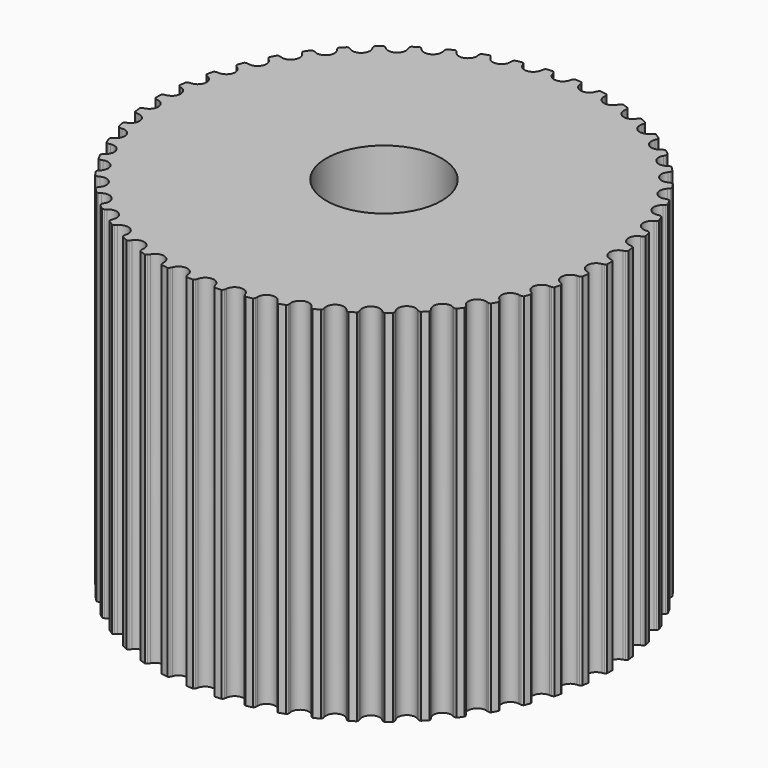
from build123d import *

# Parameters (mm, degrees)
F0_R     = 4
F1_DEPTH = 25


# Not quite as in the source:
# - ends of sketch curves that miss each other by under 0.0002 mm in the source are joined


with BuildPart() as f1:
    # F0 (on Top) → F1 (new body)
    with BuildSketch(Plane.XY):
        with BuildLine():
            ThreePointArc((5.0538548701, 14.8313976165), (4.8338819161, 14.9042559245), (4.6129350386, 14.9741051251))
            ThreePointArc((4.6129350386, 14.9741051251), (4.5441993324, 14.946267968), (4.4878171315, 14.8980958886))
            ThreePointArc((4.4878171315, 14.8980958886), (4.4420209944, 14.8370934455), (4.4036843047, 14.7711473513))
            ThreePointArc((4.4036843047, 14.7711473513), (3.7022053294, 14.453002295), (3.2407613785, 15.0697349868))
            ThreePointArc((3.2407613785, 15.0697349868), (3.2389362265, 15.1459926578), (3.2281934751, 15.2215118936))
            ThreePointArc((3.2281934751, 15.2215118936), (3.201998612, 15.2906625624), (3.1551368112, 15.3478637858))
            ThreePointArc((3.1551368112, 15.3478637858), (2.9277664974, 15.3925774546), (2.699806991, 15.4341839489))
            ThreePointArc((2.699806991, 15.4341839489), (2.6351025722, 15.3979510096), (2.5852026476, 15.3430922294))
            ThreePointArc((2.5852026476, 15.3430922294), (2.5474139332, 15.2768308289), (2.5176449061, 15.2066000335))
            ThreePointArc((2.5176449061, 15.2066000335), (1.8615708966, 14.8030459697), (1.3264687832, 15.3570810714))
            ThreePointArc((1.3264687832, 15.3570810714), (1.315100082, 15.432508655), (1.2949769217, 15.5060859735))
            ThreePointArc((1.2949769217, 15.5060859735), (1.2603213274, 15.5714077424), (1.2066603566, 15.622284525))
            ThreePointArc((1.2066603566, 15.622284525), (0.9754784824, 15.6381481518), (0.7441019834, 15.6508556551))
            ThreePointArc((0.7441019834, 15.6508556551), (0.684448921, 15.6067992893), (0.6418182175, 15.5461188946))
            ThreePointArc((0.6418182175, 15.5461188946), (0.6126318129, 15.4756440547), (0.5918997543, 15.4022360541))
            ThreePointArc((0.5918997543, 15.4022360541), (-0.008422, 14.919636), (-0.6087438986, 15.4022360223))
            ThreePointArc((-0.6087438986, 15.4022360223), (-0.6294758129, 15.4756440547), (-0.6586618609, 15.5461190674))
            ThreePointArc((-0.6586618609, 15.5461190674), (-0.7012312489, 15.6065826918), (-0.7608459985, 15.6503330029))
            ThreePointArc((-0.7608459985, 15.6503330029), (-0.9921926068, 15.6370972346), (-1.2233370313, 15.6207054025))
            ThreePointArc((-1.2233370313, 15.6207054025), (-1.2769989996, 15.569519629), (-1.3116886862, 15.5039742317))
            ThreePointArc((-1.3116886862, 15.5039742317), (-1.33181118, 15.4303971915), (-1.3431793008, 15.3549700274))
            ThreePointArc((-1.3431793008, 15.3549700274), (-1.8782818966, 14.8009349697), (-2.5343560792, 15.2044889718))
            ThreePointArc((-2.5343560792, 15.2044889718), (-2.5641249332, 15.2747198289), (-2.6019136975, 15.3409811969))
            ThreePointArc((-2.6019136975, 15.3409811969), (-2.6517255298, 15.3956328998), (-2.7163538339, 15.4315664618))
            ThreePointArc((-2.7163538339, 15.4315664618), (-2.9442174772, 15.3894389341), (-3.1714848475, 15.3442062603))
            ThreePointArc((-3.1714848475, 15.3442062603), (-3.2183068506, 15.2866986193), (-3.2445078833, 15.2173229763))
            ThreePointArc((-3.2445078833, 15.2173229763), (-3.2552512183, 15.1418037568), (-3.2570761686, 15.0655459941))
            ThreePointArc((-3.2570761686, 15.0655459941), (-3.7185201109, 14.4488133511), (-4.4199997516, 14.7669576202))
            ThreePointArc((-4.4199997516, 14.7669576202), (-4.4583356914, 14.8329039882), (-4.504131298, 14.8939067477))
            ThreePointArc((-4.504131298, 14.8939067477), (-4.5603999736, 14.9418840659), (-4.6290219304, 14.9694343117))
            ThreePointArc((-4.6290219304, 14.9694343117), (-4.8498095032, 14.8990807668), (-5.0696161514, 14.8257204436))
            ThreePointArc((-5.0696161514, 14.8257204436), (-5.1088617324, 14.7627975058), (-5.1261608376, 14.6906849879))
            ThreePointArc((-5.1261608376, 14.6906849879), (-5.1273535974, 14.6144149758), (-5.1196065751, 14.5385300687))
            ThreePointArc((-5.1196065751, 14.5385300687), (-5.5001148623, 13.8688261233), (-6.2359372486, 14.0965428322))
            ThreePointArc((-6.2359372486, 14.0965428322), (-6.2822362135, 14.1571640234), (-6.3353161345, 14.2119458535))
            ThreePointArc((-6.3353161345, 14.2119458535), (-6.3971546722, 14.2524927401), (-6.4686889983, 14.2712250176))
            ThreePointArc((-6.4686889983, 14.2712250176), (-6.6789174057, 14.1737545132), (-6.8877958964, 14.0734237881))
            ThreePointArc((-6.8877958964, 14.0734237881), (-6.918845823, 14.0060783452), (-6.9269704732, 13.9323659757))
            ThreePointArc((-6.9269704732, 13.9323659757), (-6.9185946899, 13.856547756), (-6.9013977373, 13.7822320773))
            ThreePointArc((-6.9013977373, 13.7822320773), (-7.1949697757, 13.0701187417), (-7.9535304625, 13.203817595))
            ThreePointArc((-7.9535304625, 13.203817595), (-8.00706254, 13.2581577974), (-8.0665899904, 13.3058550135))
            ThreePointArc((-8.0665899904, 13.3058550135), (-8.1330222057, 13.3383321973), (-8.2063400351, 13.3479511062))
            ThreePointArc((-8.2063400351, 13.3479511062), (-8.402694302, 13.2248996356), (-8.5973508141, 13.0991807164))
            ThreePointArc((-8.5973508141, 13.0991807164), (-8.6197156177, 13.0284751976), (-8.6185378436, 12.954326028))
            ThreePointArc((-8.6185378436, 12.954326028), (-8.6007257896, 12.8801553087), (-8.5743502072, 12.8085809095))
            ThreePointArc((-8.5743502072, 12.8085809095), (-8.7763549932, 12.0652885559), (-9.5456911317, 12.1028598516))
            ThreePointArc((-9.5456911317, 12.1028598516), (-9.6056123132, 12.1500616883), (-9.6706484989, 12.1899220673))
            ThreePointArc((-9.6706484989, 12.1899220673), (-9.740627088, 12.213816696), (-9.814571967, 12.214170792))
            ThreePointArc((-9.814571967, 12.214170792), (-9.9939559602, 12.0674808947), (-10.171321105, 11.9183561232))
            ThreePointArc((-10.171321105, 11.9183561232), (-10.1846477481, 11.8454047013), (-10.174185817, 11.7719877449))
            ThreePointArc((-10.174185817, 11.7719877449), (-10.1472175675, 11.7006345891), (-10.1120794197, 11.6329303458))
            ThreePointArc((-10.1120794197, 11.6329303458), (-10.219332575, 10.8701815734), (-10.9873108533, 10.8110332144))
            ThreePointArc((-10.9873108533, 10.8110332144), (-11.0526756486, 10.8503529134), (-11.1221950662, 10.881747827))
            ThreePointArc((-11.1221950662, 10.881747827), (-11.1946168625, 10.8966831818), (-11.2680231697, 10.8877665837))
            ThreePointArc((-11.2680231697, 10.8877665837), (-11.4276069367, 10.7197501445), (-11.5848828695, 10.549571881))
            ThreePointArc((-11.5848828695, 10.549571881), (-11.5889613448, 10.4755251639), (-11.5693801663, 10.4039979241))
            ThreePointArc((-11.5693801663, 10.4039979241), (-11.5336822713, 10.3365870506), (-11.4903354338, 10.2738206612))
            ThreePointArc((-11.4903354338, 10.2738206612), (-11.5011451489, 9.5036439453), (-12.2556548017, 9.348709386))
            ThreePointArc((-12.2556548017, 9.348709386), (-12.3254316288, 9.3795265133), (-12.3983370749, 9.4019606939))
            ThreePointArc((-12.3983370749, 9.4019606939), (-12.4720599509, 9.4077023581), (-12.5437703187, 9.3896557359))
            ThreePointArc((-12.5437703187, 9.3896557359), (-12.681037629, 9.202962339), (-12.8157446424, 9.0144137482))
            ThreePointArc((-12.8157446424, 9.0144137482), (-12.8105102139, 8.9404404944), (-12.7821190203, 8.8719319874))
            ThreePointArc((-12.7821190203, 8.8719319874), (-12.7382537529, 8.8095267396), (-12.6873820393, 8.7526879605))
            ThreePointArc((-12.6873820393, 8.7526879605), (-12.6015775657, 7.9872298991), (-13.3307188206, 7.738951493))
            ThreePointArc((-13.3307188206, 7.738951493), (-13.4038082989, 7.7607801426), (-13.4789510081, 7.7738999297))
            ThreePointArc((-13.4789510081, 7.7738999297), (-13.5528120665, 7.7703559957), (-13.621694978, 7.7434639629))
            ThreePointArc((-13.621694978, 7.7434639629), (-13.7344808688, 7.5410388275), (-13.8444943275, 7.3370936431))
            ThreePointArc((-13.8444943275, 7.3370936431), (-13.830030191, 7.2643597641), (-13.7932762752, 7.1999497776))
            ThreePointArc((-13.7932762752, 7.1999497776), (-13.741935461, 7.1435344537), (-13.6843411261, 7.0935198363))
            ThreePointArc((-13.6843411261, 7.0935198363), (-13.5032758231, 6.3448511641), (-14.1955500939, 6.0071445862))
            ThreePointArc((-14.1955500939, 6.0071445862), (-14.2707991813, 6.0196415185), (-14.3469940004, 6.0232400332))
            ThreePointArc((-14.3469940004, 6.0232400332), (-14.419828172, 6.0104665165), (-14.4847971498, 5.9751531931))
            ThreePointArc((-14.4847971498, 5.9751531931), (-14.5713237993, 5.7601890844), (-14.6549084852, 5.5440641838))
            ThreePointArc((-14.6549084852, 5.5440641838), (-14.6314415623, 5.4737160221), (-14.5869047411, 5.4144202694))
            ThreePointArc((-14.5869047411, 5.4144202694), (-14.5288983722, 5.3648846331), (-14.4654900012, 5.3224829979))
            ThreePointArc((-14.4654900012, 5.3224829979), (-14.1920195403, 4.6024115579), (-14.8365090025, 4.1806029748))
            ThreePointArc((-14.8365090025, 4.1806029748), (-14.9127305279, 4.1835697694), (-14.9887750296, 4.1775902142))
            ThreePointArc((-14.9887750296, 4.1775902142), (-15.0594343442, 4.1557890775), (-15.1194655457, 4.1126115454))
            ThreePointArc((-15.1194655457, 4.1126115454), (-15.1783673815, 3.8884970823), (-15.2342054342, 3.6636001047))
            ThreePointArc((-15.2342054342, 3.6636001047), (-15.2021067766, 3.5967482868), (-15.1504897798, 3.5435022959))
            ThreePointArc((-15.1504897798, 3.5435022959), (-15.0867323168, 3.5016267428), (-15.0185092191, 3.4675064891))
            ThreePointArc((-15.0185092191, 3.4675064891), (-14.6569456659, 2.7873884892), (-15.2434870034, 2.2881301223))
            ThreePointArc((-15.2434870034, 2.2881301223), (-15.3194794639, 2.2815203887), (-15.3941750247, 2.2660570919))
            ThreePointArc((-15.3941750247, 2.2660570919), (-15.4615445837, 2.2355715421), (-15.515690764, 2.1852105923))
            ThreePointArc((-15.515690764, 2.1852105923), (-15.546039204, 1.95548092), (-15.5732498745, 1.725358986))
            ThreePointArc((-15.5732498745, 1.725358986), (-15.5330257102, 1.6630571566), (-15.4751419402, 1.6167001059))
            ThreePointArc((-15.4751419402, 1.6167001059), (-15.4066385356, 1.583146357), (-15.3346770307, 1.5578458931))
            ThreePointArc((-15.3346770307, 1.5578458931), (-14.8907239251, 0.9284060096), (-15.4100659026, 0.3595713715))
            ThreePointArc((-15.4100659026, 0.3595713715), (-15.4846311438, 0.3434894327), (-15.5568000022, 0.3187860053))
            ThreePointArc((-15.5568000022, 0.3187860053), (-15.6198171565, 0.2800971716), (-15.667224202, 0.2233471194))
            ThreePointArc((-15.667224202, 0.2233471194), (-15.6685409464, -0.0083743057), (-15.666695131, -0.2400920019))
            ThreePointArc((-15.666695131, -0.2400920019), (-15.6189792515, -0.2968609065), (-15.5557417451, -0.3355973772))
            ThreePointArc((-15.5557417451, -0.3355973772), (-15.4835735155, -0.3603006073), (-15.4090088937, -0.3763823142))
            ThreePointArc((-15.4090088937, -0.3763823142), (-14.889665926, -0.9452169962), (-15.3336199522, -1.5746571665))
            ThreePointArc((-15.3336199522, -1.5746571665), (-15.4055809789, -1.5999575427), (-15.4740840038, -1.6335109932))
            ThreePointArc((-15.4740840038, -1.6335109932), (-15.5317555659, -1.6797932906), (-15.5716765135, -1.7420377779))
            ThreePointArc((-15.5716765135, -1.7420377779), (-15.5439399716, -1.9720969632), (-15.5130668126, -2.2017559735))
            ThreePointArc((-15.5130668126, -2.2017559735), (-15.458612789, -2.2520973071), (-15.3910189313, -2.2826027445))
            ThreePointArc((-15.3910189313, -2.2826027445), (-15.3163234361, -2.2980662463), (-15.2403309956, -2.3046758423))
            ThreePointArc((-15.2403309956, -2.3046758423), (-14.6537896659, -2.8039344892), (-15.0153528268, -3.4840534039))
            ThreePointArc((-15.0153528268, -3.4840534039), (-15.0835759692, -3.5181725426), (-15.1473335858, -3.5600472129))
            ThreePointArc((-15.1473335858, -3.5600472129), (-15.1987489134, -3.6131932305), (-15.2305535043, -3.6799501439))
            ThreePointArc((-15.2305535043, -3.6799501439), (-15.1742017793, -3.9047182734), (-15.1147881975, -4.1286967812))
            ThreePointArc((-15.1147881975, -4.1286967812), (-15.0544545219, -4.1718167767), (-14.9835700248, -4.1936101796))
            ThreePointArc((-14.9835700248, -4.1936101796), (-14.9075255279, -4.1995897694), (-14.8313040188, -4.1966228082))
            ThreePointArc((-14.8313040188, -4.1966228082), (-14.1868146735, -4.6184311478), (-14.4602841651, -5.3385027186))
            ThreePointArc((-14.4602841651, -5.3385027186), (-14.5236930285, -5.3809043728), (-14.5816999026, -5.4304401013))
            ThreePointArc((-14.5816999026, -5.4304401013), (-14.6260492492, -5.4896104411), (-14.6492361553, -5.5598269754))
            ThreePointArc((-14.6492361553, -5.5598269754), (-14.5651581949, -5.7757608344), (-14.4781410205, -5.9905270085))
            ThreePointArc((-14.4781410205, -5.9905270085), (-14.4128783592, -6.0257443518), (-14.3398220082, -6.0384817165))
            ThreePointArc((-14.3398220082, -6.0384817165), (-14.2636271813, -6.0348825185), (-14.1883780616, -6.0223857287))
            ThreePointArc((-14.1883780616, -6.0223857287), (-13.4961039059, -6.3600929882), (-13.677168659, -7.1087614426))
            ThreePointArc((-13.677168659, -7.1087614426), (-13.7347629645, -7.1587759687), (-13.7861039068, -7.2151910753))
            ThreePointArc((-13.7861039068, -7.2151910753), (-13.8226881352, -7.2794529438), (-13.8368918149, -7.3520219746))
            ThreePointArc((-13.8368918149, -7.3520219746), (-13.726412769, -7.5557153361), (-13.6131645058, -7.7578817187))
            ThreePointArc((-13.6131645058, -7.7578817187), (-13.5440023262, -7.7846419987), (-13.4699249773, -7.788122198))
            ThreePointArc((-13.4699249773, -7.788122198), (-13.3947821363, -7.7750028685), (-13.3216928545, -7.7531734))
            ThreePointArc((-13.3216928545, -7.7531734), (-12.592552504, -8.0014519963), (-12.6783560356, -8.7669099641))
            ThreePointArc((-12.6783560356, -8.7669099641), (-12.7292278849, -8.8237486471), (-12.7730934307, -8.8861537336))
            ThreePointArc((-12.7730934307, -8.8861537336), (-12.801334547, -8.9544947169), (-12.8063308647, -9.0282719872))
            ThreePointArc((-12.8063308647, -9.0282719872), (-12.6711936702, -9.2165123799), (-12.5335000743, -9.4028910557))
            ThreePointArc((-12.5335000743, -9.4028910557), (-12.4615291151, -9.4207717741), (-12.3875999414, -9.4149402395))
            ThreePointArc((-12.3875999414, -9.4149402395), (-12.3146946288, -9.3925055133), (-12.2449180268, -9.3616879479))
            ThreePointArc((-12.2449180268, -9.3616879479), (-11.4904081489, -9.5166229453), (-11.4795980172, -10.2867999865))
            ThreePointArc((-11.4795980172, -10.2867999865), (-11.5229452713, -10.3495660506), (-11.5586434111, -10.4169768123))
            ThreePointArc((-11.5586434111, -10.4169768123), (-11.5780965344, -10.4883184077), (-11.5738065918, -10.5621401325))
            ThreePointArc((-11.5738065918, -10.5621401325), (-11.4161417319, -10.7319585543), (-11.2561747164, -10.8996097256))
            ThreePointArc((-11.2561747164, -10.8996097256), (-11.1825310932, -10.9083297135), (-11.1099161508, -10.8932786059))
            ThreePointArc((-11.1099161508, -10.8932786059), (-11.0403966486, -10.8618839134), (-10.9750321796, -10.8225637377))
            ThreePointArc((-10.9750321796, -10.8225637377), (-10.2070536544, -10.8817114989), (-10.0998003881, -11.6444607687))
            ThreePointArc((-10.0998003881, -11.6444607687), (-10.1349382684, -11.7121649196), (-10.1619059639, -11.7835180113))
            ThreePointArc((-10.1619059639, -11.7835180113), (-10.1722646357, -11.8567350859), (-10.1587561762, -11.9294370635))
            ThreePointArc((-10.1587561762, -11.9294370635), (-9.9810515294, -12.0781566272), (-9.8013335612, -12.2244366992))
            ThreePointArc((-9.8013335612, -12.2244366992), (-9.7271768114, -12.2238569185), (-9.6570207455, -12.1998234759))
            ThreePointArc((-9.6570207455, -12.1998234759), (-9.5919847883, -12.1599630193), (-9.532064145, -12.1127608367))
            ThreePointArc((-9.532064145, -12.1127608367), (-8.7627283639, -12.0751892866), (-8.5607226129, -12.8184811691))
            ThreePointArc((-8.5607226129, -12.8184811691), (-8.5870975719, -12.8900555907), (-8.6049097911, -12.9642260374))
            ThreePointArc((-8.6049097911, -12.9642260374), (-8.6060103202, -13.0381640872), (-8.5834966058, -13.108599799))
            ThreePointArc((-8.5834966058, -13.108599799), (-8.388553235, -13.2338732494), (-8.1919185578, -13.3564752799))
            ThreePointArc((-8.1919185578, -13.3564752799), (-8.1184199503, -13.3466067448), (-8.0518291493, -13.3139697895))
            ThreePointArc((-8.0518291493, -13.3139697895), (-7.9923012608, -13.2662725454), (-7.9387688944, -13.2119320925))
            ThreePointArc((-7.9387688944, -13.2119320925), (-7.1802084461, -13.0782339229), (-6.8866369815, -13.7903470055))
            ThreePointArc((-6.8866369815, -13.7903470055), (-6.9038336942, -13.8646627813), (-6.9122093766, -13.940481032))
            ThreePointArc((-6.9122093766, -13.940481032), (-6.9040346955, -14.0139738874), (-6.8728705786, -14.0810323934))
            ThreePointArc((-6.8728705786, -14.0810323934), (-6.6637629881, -14.1808852229), (-6.4533128154, -14.2778755922))
            ThreePointArc((-6.4533128154, -14.2778755922), (-6.3816304907, -14.2588723625), (-6.3196552888, -14.2181466853))
            ThreePointArc((-6.3196552888, -14.2181466853), (-6.2665744539, -14.1633653025), (-6.220274882, -14.1027440796))
            ThreePointArc((-6.220274882, -14.1027440796), (-5.4844528623, -13.8750271233), (-5.1039450327, -14.5447309947))
            ThreePointArc((-5.1039450327, -14.5447309947), (-5.1116925956, -14.6206159331), (-5.1104996151, -14.6968860458))
            ThreePointArc((-5.1104996151, -14.6968860458), (-5.0931771747, -14.7687745105), (-5.0538540874, -14.8313980771))
            ThreePointArc((-5.0538540874, -14.8313980771), (-4.833881011, -14.9042562174), (-4.6129341256, -14.9741054069))
            ThreePointArc((-4.6129341256, -14.9741054069), (-4.5441983324, -14.946267968), (-4.4878161315, -14.8980958886))
            ThreePointArc((-4.4878161315, -14.8980958886), (-4.4420206914, -14.8370929882), (-4.4036841013, -14.7711469488))
            ThreePointArc((-4.4036841013, -14.7711469488), (-3.7022043125, -14.4530022993), (-3.2407603797, -15.0697350216))
            ThreePointArc((-3.2407603797, -15.0697350216), (-3.2389362183, -15.1459927568), (-3.2281934356, -15.2215120883))
            ThreePointArc((-3.2281934356, -15.2215120883), (-3.201997612, -15.2906625624), (-3.1551358112, -15.3478637858))
            ThreePointArc((-3.1551358112, -15.3478637858), (-2.9277659812, -15.3925773628), (-2.6998069612, -15.4341837786))
            ThreePointArc((-2.6998069612, -15.4341837786), (-2.63510194, -15.397951302), (-2.5852016476, -15.3430922294))
            ThreePointArc((-2.5852016476, -15.3430922294), (-2.5474129332, -15.2768308289), (-2.5176439061, -15.2066000335))
            ThreePointArc((-2.5176439061, -15.2066000335), (-1.8615699417, -14.803045964), (-1.3264677915, -15.357080981))
            ThreePointArc((-1.3264677915, -15.357080981), (-1.3150991245, -15.432508454), (-1.294976024, -15.5060856704))
            ThreePointArc((-1.294976024, -15.5060856704), (-1.2603210771, -15.5714080717), (-1.2066596723, -15.6222849898))
            ThreePointArc((-1.2066596723, -15.6222849898), (-0.9754779809, -15.638148121), (-0.7441019811, -15.6508556072))
            ThreePointArc((-0.7441019811, -15.6508556072), (-0.684448384, -15.6067997635), (-0.6418174078, -15.546119287))
            ThreePointArc((-0.6418174078, -15.546119287), (-0.6126317777, -15.4756439532), (-0.5918997081, -15.4022358442))
            ThreePointArc((-0.5918997081, -15.4022358442), (0.0084221074, -14.919636), (0.6087438986, -15.4022360223))
            ThreePointArc((0.6087438986, -15.4022360223), (0.6294767062, -15.4756437472), (0.6586626706, -15.546118675))
            ThreePointArc((0.6586626706, -15.546118675), (0.7012315608, -15.6065830099), (0.7608467926, -15.6503334072))
            ThreePointArc((0.7608467926, -15.6503334072), (0.9921936068, -15.6370972346), (1.2233380313, -15.6207054025))
            ThreePointArc((1.2233380313, -15.6207054025), (1.2769993451, -15.5695191725), (1.3116887886, -15.5039739286))
            ThreePointArc((1.3116887886, -15.5039739286), (1.33181218, -15.4303971915), (1.3431803008, -15.3549700274))
            ThreePointArc((1.3431803008, -15.3549700274), (1.8782819417, -14.800934964), (2.5343560792, -15.2044889718))
            ThreePointArc((2.5343560792, -15.2044889718), (2.5641249332, -15.2747198289), (2.6019136975, -15.3409811969))
            ThreePointArc((2.6019136975, -15.3409811969), (2.6517255298, -15.3956328998), (2.7163538339, -15.4315664618))
            ThreePointArc((2.7163538339, -15.4315664618), (2.9442175129, -15.3894391192), (3.1714848883, -15.344206458))
            ThreePointArc((3.1714848883, -15.344206458), (3.2183076641, -15.2866989433), (3.2445088833, -15.2173229763))
            ThreePointArc((3.2445088833, -15.2173229763), (3.2552512251, -15.1418036751), (3.2570761698, -15.0655460289))
            ThreePointArc((3.2570761698, -15.0655460289), (3.7185203125, -14.4488132993), (4.419999955, -14.7669580227))
            ThreePointArc((4.419999955, -14.7669580227), (4.4583366914, -14.8329039882), (4.504132298, -14.8939067477))
            ThreePointArc((4.504132298, -14.8939067477), (4.5604006677, -14.9418844857), (4.6290228829, -14.9694345244))
            ThreePointArc((4.6290228829, -14.9694345244), (4.8498100533, -14.8990809135), (5.0696162558, -14.8257207494))
            ThreePointArc((5.0696162558, -14.8257207494), (5.1088617324, -14.7627975058), (5.1261608376, -14.6906849879))
            ThreePointArc((5.1261608376, -14.6906849879), (5.1273545956, -14.6144149331), (5.1196075496, -14.5385299111))
            ThreePointArc((5.1196075496, -14.5385299111), (5.5001148623, -13.8688261233), (6.2359372486, -14.0965428322))
            ThreePointArc((6.2359372486, -14.0965428322), (6.2822364539, -14.1571643025), (6.3353166773, -14.2119463516))
            ThreePointArc((6.3353166773, -14.2119463516), (6.3971552173, -14.252492538), (6.4686890071, -14.2712249242))
            ThreePointArc((6.4686890071, -14.2712249242), (6.6789175879, -14.1737548992), (6.8877960893, -14.0734241826))
            ThreePointArc((6.8877960893, -14.0734241826), (6.9188467482, -14.0060786145), (6.9269714732, -13.9323659757))
            ThreePointArc((6.9269714732, -13.9323659757), (6.9185956662, -13.8565476169), (6.9013986577, -13.7822318065))
            ThreePointArc((6.9013986577, -13.7822318065), (7.1949708994, -13.0701186737), (7.9535314625, -13.203817595))
            ThreePointArc((7.9535314625, -13.203817595), (8.0070627845, -13.2581580181), (8.0665899904, -13.3058550135))
            ThreePointArc((8.0665899904, -13.3058550135), (8.1330228152, -13.3383320796), (8.2063410351, -13.3479511062))
            ThreePointArc((8.2063410351, -13.3479511062), (8.402695302, -13.2248996356), (8.5973518141, -13.0991807164))
            ThreePointArc((8.5973518141, -13.0991807164), (8.6197166304, -13.0284751105), (8.6185388126, -12.9543258546))
            ThreePointArc((8.6185388126, -12.9543258546), (8.6007258477, -12.8801555002), (8.5743503673, -12.8085812763))
            ThreePointArc((8.5743503673, -12.8085812763), (8.7763559932, -12.0652885559), (9.5456921317, -12.1028598516))
            ThreePointArc((9.5456921317, -12.1028598516), (9.6056129818, -12.1500621541), (9.6706492764, -12.1899224832))
            ThreePointArc((9.6706492764, -12.1899224832), (9.7406280098, -12.2138168513), (9.8145729424, -12.2141706372))
            ThreePointArc((9.8145729424, -12.2141706372), (9.9939565527, -12.0674804034), (10.1713216841, -11.9183556295))
            ThreePointArc((10.1713216841, -11.9183556295), (10.1846477484, -11.8454046827), (10.1741859059, -11.7719880294))
            ThreePointArc((10.1741859059, -11.7719880294), (10.1472184631, -11.7006343554), (10.1120801576, -11.6329299061))
            ThreePointArc((10.1120801576, -11.6329299061), (10.2193337616, -10.8701813982), (10.9873118533, -10.8110332144))
            ThreePointArc((10.9873118533, -10.8110332144), (11.052676235, -10.8503526966), (11.122195194, -10.8817474932))
            ThreePointArc((11.122195194, -10.8817474932), (11.1946173422, -10.8966832016), (11.2680240918, -10.8877663156))
            ThreePointArc((11.2680240918, -10.8877663156), (11.4276079367, -10.7197501445), (11.5848838695, -10.549571881))
            ThreePointArc((11.5848838695, -10.549571881), (11.5889623448, -10.4755251639), (11.5693811663, -10.4039979241))
            ThreePointArc((11.5693811663, -10.4039979241), (11.5336825389, -10.3365874912), (11.4903358127, -10.2738211463))
            ThreePointArc((11.4903358127, -10.2738211463), (11.5011458654, -9.5036442879), (12.2556550105, -9.3487089795))
            ThreePointArc((12.2556550105, -9.3487089795), (12.3254320838, -9.3795266831), (12.3983380184, -9.4019609246))
            ThreePointArc((12.3983380184, -9.4019609246), (12.4720609509, -9.4077023581), (12.5437713187, -9.3896557359))
            ThreePointArc((12.5437713187, -9.3896557359), (12.68103846, -9.2029625721), (12.8157453109, -9.0144142189))
            ThreePointArc((12.8157453109, -9.0144142189), (12.8105112242, -8.9404405384), (12.7821200203, -8.8719319874))
            ThreePointArc((12.7821200203, -8.8719319874), (12.7382547529, -8.8095267396), (12.6873830393, -8.7526879605))
            ThreePointArc((12.6873830393, -8.7526879605), (12.6015785657, -7.9872298991), (13.3307198206, -7.738951493))
            ThreePointArc((13.3307198206, -7.738951493), (13.4038092989, -7.7607801426), (13.4789520081, -7.7738999297))
            ThreePointArc((13.4789520081, -7.7738999297), (13.5528126457, -7.7703560855), (13.6216952374, -7.7434644012))
            ThreePointArc((13.6216952374, -7.7434644012), (13.7344816377, -7.541039249), (13.8444951078, -7.3370940572))
            ThreePointArc((13.8444951078, -7.3370940572), (13.830030301, -7.2643600585), (13.7932766703, -7.1999502664))
            ThreePointArc((13.7932766703, -7.1999502664), (13.7419356857, -7.1435346733), (13.6843411261, -7.0935198363))
            ThreePointArc((13.6843411261, -7.0935198363), (13.5032769918, -6.3448508057), (14.1955510939, -6.0071445862))
            ThreePointArc((14.1955510939, -6.0071445862), (14.2707996661, -6.01964157), (14.3469940004, -6.0232400332))
            ThreePointArc((14.3469940004, -6.0232400332), (14.419828327, -6.0104668114), (14.4847975257, -5.9751536774))
            ThreePointArc((14.4847975257, -5.9751536774), (14.5713238643, -5.7601889196), (14.6549086107, -5.5440638525))
            ThreePointArc((14.6549086107, -5.5440638525), (14.6314425623, -5.4737160221), (14.5869057411, -5.4144202694))
            ThreePointArc((14.5869057411, -5.4144202694), (14.5288990285, -5.3648843728), (14.4654902574, -5.3224825614))
            ThreePointArc((14.4654902574, -5.3224825614), (14.1920195403, -4.6024115579), (14.8365090025, -4.1806029748))
            ThreePointArc((14.8365090025, -4.1806029748), (14.9127310304, -4.1835697793), (14.9887760296, -4.1775902142))
            ThreePointArc((14.9887760296, -4.1775902142), (15.0594351042, -4.1557886997), (15.1194660454, -4.1126110454))
            ThreePointArc((15.1194660454, -4.1126110454), (15.1783674428, -3.8884968424), (15.2342054891, -3.6635998768))
            ThreePointArc((15.2342054891, -3.6635998768), (15.2021075472, -3.5967479577), (15.1504901363, -3.5435018169))
            ThreePointArc((15.1504901363, -3.5435018169), (15.0867325709, -3.5016263133), (15.0185093744, -3.4675061269))
            ThreePointArc((15.0185093744, -3.4675061269), (14.656946752, -2.7873880378), (15.2434880034, -2.2881301223))
            ThreePointArc((15.2434880034, -2.2881301223), (15.3194804361, -2.2815202463), (15.3941759572, -2.266056841))
            ThreePointArc((15.3941759572, -2.266056841), (15.4615452407, -2.235571105), (15.5156911394, -2.1852101081))
            ThreePointArc((15.5156911394, -2.1852101081), (15.546040204, -1.95548092), (15.5732508745, -1.725358986))
            ThreePointArc((15.5732508745, -1.725358986), (15.5330267102, -1.6630571566), (15.4751429402, -1.6167001059))
            ThreePointArc((15.4751429402, -1.6167001059), (15.4066393804, -1.5831467109), (15.3346779546, -1.5578461582))
            ThreePointArc((15.3346779546, -1.5578461582), (14.8907249251, -0.9284060096), (15.4100669026, -0.3595713715))
            ThreePointArc((15.4100669026, -0.3595713715), (15.484631698, -0.3434895566), (15.5568001456, -0.3187863558))
            ThreePointArc((15.5568001456, -0.3187863558), (15.6198178064, -0.2800974742), (15.667225202, -0.2233471194))
            ThreePointArc((15.667225202, -0.2233471194), (15.6685409464, 0.0083743046), (15.6666951312, 0.2400919871))
            ThreePointArc((15.6666951312, 0.2400919871), (15.6189797964, 0.2968604375), (15.5557426016, 0.3355970266))
            ThreePointArc((15.5557426016, 0.3355970266), (15.4835739614, 0.3603004834), (15.4090088937, 0.3763823142))
            ThreePointArc((15.4090088937, 0.3763823142), (14.8896669251, 0.9452170096), (15.3336200283, 1.5746569014))
            ThreePointArc((15.3336200283, 1.5746569014), (15.4055815356, 1.599957357), (15.4740850038, 1.6335109932))
            ThreePointArc((15.4740850038, 1.6335109932), (15.5317559897, 1.6797937619), (15.5716766711, 1.7420381422))
            ThreePointArc((15.5716766711, 1.7420381422), (15.5439409716, 1.9720969632), (15.5130678126, 2.2017559735))
            ThreePointArc((15.5130678126, 2.2017559735), (15.4586134483, 2.2520968704), (15.3910198638, 2.2826024936))
            ThreePointArc((15.3910198638, 2.2826024936), (15.3163239416, 2.2980663188), (15.2403309964, 2.3046758704))
            ThreePointArc((15.2403309964, 2.3046758704), (14.6537906584, 2.8039345287), (15.0153529821, 3.4840530417))
            ThreePointArc((15.0153529821, 3.4840530417), (15.0835763168, 3.5181727428), (15.1473342293, 3.5600476919))
            ThreePointArc((15.1473342293, 3.5600476919), (15.1987498339, 3.613193116), (15.2305544266, 3.6799498762))
            ThreePointArc((15.2305544266, 3.6799498762), (15.1742027169, 3.9047185152), (15.1147891283, 4.128697035))
            ThreePointArc((15.1147891283, 4.128697035), (15.0544552038, 4.1718169341), (14.9835710248, 4.1936101796))
            ThreePointArc((14.9835710248, 4.1936101796), (14.9075260231, 4.1995897596), (14.8313040188, 4.1966228082))
            ThreePointArc((14.8313040188, 4.1966228082), (14.1868145403, 4.6184315579), (14.4602849089, 5.3385031551))
            ThreePointArc((14.4602849089, 5.3385031551), (14.523693741, 5.3809041551), (14.5817003827, 5.4304396017))
            ThreePointArc((14.5817003827, 5.4304396017), (14.6260500823, 5.4896101215), (14.6492371553, 5.5598269754))
            ThreePointArc((14.6492371553, 5.5598269754), (14.5651583312, 5.7757604913), (14.4781411663, 5.9905266556))
            ThreePointArc((14.4781411663, 5.9905266556), (14.4128788868, 6.0257445156), (14.3398220084, 6.038481728))
            ThreePointArc((14.3398220084, 6.038481728), (14.2636276661, 6.03488257), (14.1883790126, 6.0223859446))
            ThreePointArc((14.1883790126, 6.0223859446), (13.4961050746, 6.3600926298), (13.6771690314, 7.1087609592))
            ThreePointArc((13.6771690314, 7.1087609592), (13.7347631893, 7.1587761883), (13.7861043019, 7.2151915641))
            ThreePointArc((13.7861043019, 7.2151915641), (13.82268825, 7.2794532531), (13.8368918159, 7.3520220057))
            ThreePointArc((13.8368918159, 7.3520220057), (13.7264128827, 7.55571513), (13.6131645058, 7.7578817187))
            ThreePointArc((13.6131645058, 7.7578817187), (13.5440028123, 7.7846418961), (13.4699259643, 7.7881223112))
            ThreePointArc((13.4699259643, 7.7881223112), (13.3947830771, 7.7750030903), (13.3216937376, 7.7531737212))
            ThreePointArc((13.3216937376, 7.7531737212), (12.5925525657, 8.0014518991), (12.678356539, 8.7669104641))
            ThreePointArc((12.678356539, 8.7669104641), (12.7292282692, 8.8237491308), (12.7730937075, 8.886154181))
            ThreePointArc((12.7730937075, 8.886154181), (12.8013355577, 8.9544947628), (12.8063318558, 9.0282720811))
            ThreePointArc((12.8063318558, 9.0282720811), (12.6711938467, 9.2165121376), (12.5335004339, 9.4028905758))
            ThreePointArc((12.5335004339, 9.4028905758), (12.4615301151, 9.4207717741), (12.3876009414, 9.4149402395))
            ThreePointArc((12.3876009414, 9.4149402395), (12.3146950838, 9.3925056831), (12.2449180268, 9.3616879479))
            ThreePointArc((12.2449180268, 9.3616879479), (11.4904088654, 9.5166232879), (11.4795990172, 10.2867999865))
            ThreePointArc((11.4795990172, 10.2867999865), (11.5229455389, 10.3495664912), (11.5586435836, 10.4169771901))
            ThreePointArc((11.5586435836, 10.4169771901), (11.5780975344, 10.4883184077), (11.5738075918, 10.5621401325))
            ThreePointArc((11.5738075918, 10.5621401325), (11.4161427319, 10.7319585543), (11.2561757164, 10.8996097256))
            ThreePointArc((11.2561757164, 10.8996097256), (11.1825315734, 10.9083297343), (11.1099161508, 10.8932786059))
            ThreePointArc((11.1099161508, 10.8932786059), (11.040397235, 10.8618836966), (10.9750331796, 10.8225637377))
            ThreePointArc((10.9750331796, 10.8225637377), (10.2070546544, 10.8817114989), (10.0998013881, 11.6444607687))
            ThreePointArc((10.0998013881, 11.6444607687), (10.1349392684, 11.7121649196), (10.1619069639, 11.7835180113))
            ThreePointArc((10.1619069639, 11.7835180113), (10.1722656357, 11.8567350859), (10.1587571762, 11.9294370635))
            ThreePointArc((10.1587571762, 11.9294370635), (9.9810521242, 12.0781561364), (9.8013341694, 12.224436211))
            ThreePointArc((9.8013341694, 12.224436211), (9.7271773768, 12.2238568443), (9.6570209679, 12.19982306))
            ThreePointArc((9.6570209679, 12.19982306), (9.5919851197, 12.1599625535), (9.5320645856, 12.1127603402))
            ThreePointArc((9.5320645856, 12.1127603402), (8.7627283639, 12.0751892866), (8.5607226129, 12.8184811691))
            ThreePointArc((8.5607226129, 12.8184811691), (8.5870985138, 12.8900553992), (8.6049107911, 12.9642260374))
            ThreePointArc((8.6049107911, 12.9642260374), (8.6060112869, 13.0381643119), (8.5834973994, 13.1086002037))
            ThreePointArc((8.5834973994, 13.1086002037), (8.3885535212, 13.2338737013), (8.1919188316, 13.3564757258))
            ThreePointArc((8.1919188316, 13.3564757258), (8.1184200817, 13.3466064813), (8.0518294839, 13.3139693176))
            ThreePointArc((8.0518294839, 13.3139693176), (7.9923015053, 13.266272766), (7.9387693284, 13.2119325881))
            ThreePointArc((7.9387693284, 13.2119325881), (7.1802094461, 13.0782339229), (6.8866379815, 13.7903470055))
            ThreePointArc((6.8866379815, 13.7903470055), (6.9038346899, 13.864662756), (6.9122103739, 13.9404809808))
            ThreePointArc((6.9122103739, 13.9404809808), (6.9040347713, 14.0139736166), (6.8728708948, 14.0810319284))
            ThreePointArc((6.8728708948, 14.0810319284), (6.6637633953, 14.1808850319), (6.4533128154, 14.2778755922))
            ThreePointArc((6.4533128154, 14.2778755922), (6.381630827, 14.2588725128), (6.3196558316, 14.2181471835))
            ThreePointArc((6.3196558316, 14.2181471835), (6.2665754539, 14.1633653025), (6.220275882, 14.1027440796))
            ThreePointArc((6.220275882, 14.1027440796), (5.4844538623, 13.8750271233), (5.1039460327, 14.5447309947))
            ThreePointArc((5.1039460327, 14.5447309947), (5.1116925974, 14.6206159758), (5.1104996206, 14.6968859717))
            ThreePointArc((5.1104996206, 14.6968859717), (5.0931781747, 14.7687745105), (5.0538548701, 14.8313976165))
        make_face()
        Circle(F0_R, mode=Mode.SUBTRACT)
    extrude(amount=F1_DEPTH)


solid = f1.part
